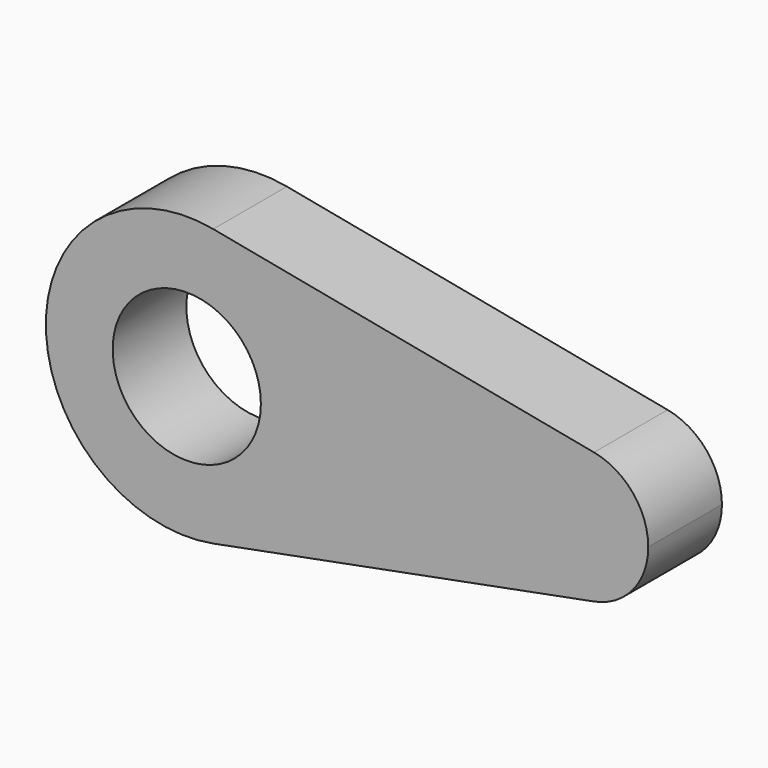
from build123d import *

# Parameters (mm, degrees)
F0_R     = 28.1638511083
F1_DEPTH = 35


# Not quite as in the source:
# - the program builds the solid bodies; features that only make, move or delete a surface that nothing else refers to are left out


with BuildPart() as f1:
    # F0 (on Front) → F1 (new body)
    with BuildSketch(Plane.XZ):
        with BuildLine():
            ThreePointArc((10.057095516, 52.6112248036), (41.2782201188, 34.1349482111), (53.5638511083, 0))
            ThreePointArc((53.5638511083, 0), (41.2782201188, -34.1349482111), (10.057095516, -52.6112248036))
            Line((10.057095516, -52.6112248036), (154.7690787877, -24.9482642185))
            ThreePointArc((154.7690787877, -24.9482642185), (124.6, 0), (154.7690787877, 24.9482642185))
            Line((154.7690787877, 24.9482642185), (10.057095516, 52.6112248036))
        make_face()
        with BuildLine():
            ThreePointArc((10.057095516, -52.6112248036), (41.2782201188, -34.1349482111), (53.5638511083, 0))
            ThreePointArc((53.5638511083, 0), (41.2782201188, 34.1349482111), (10.057095516, 52.6112248036))
            ThreePointArc((10.057095516, 52.6112248036), (-53.5638511083, 0), (10.057095516, -52.6112248036))
        make_face()
        Circle(F0_R, mode=Mode.SUBTRACT)
        with BuildLine():
            ThreePointArc((175.4, 0), (169.5741487836, 16.1868063372), (154.7690787877, 24.9482642185))
            ThreePointArc((154.7690787877, 24.9482642185), (124.6, 0), (154.7690787877, -24.9482642185))
            ThreePointArc((154.7690787877, -24.9482642185), (169.5741487836, -16.1868063372), (175.4, 0))
        make_face()
    extrude(amount=F1_DEPTH)


solid = f1.part
